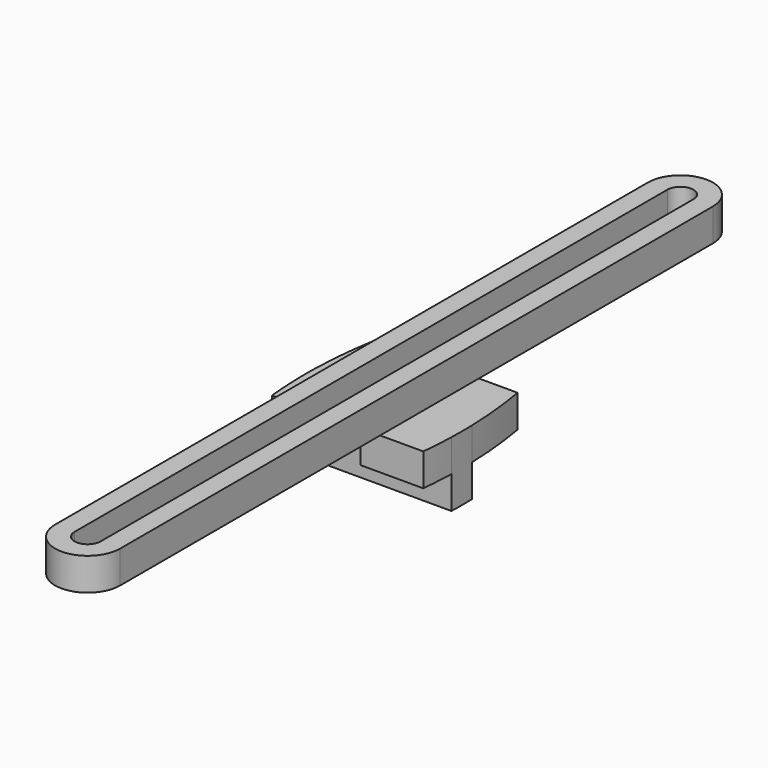
from build123d import *

# Parameters (mm, degrees)
F0_W     = 3
F0_H     = 10
F0_H_2   = 5
F1_DEPTH = 5
F2_START = -5
F2_DEPTH = 5
F3_DEPTH = 5


with BuildPart() as f1:
    # F0 (on Top) → F1 (new body)
    with BuildSketch(Plane.XY):
        with Locations((3.5, 7)):
            Rectangle(F0_W, F0_H)
        with BuildLine():
            Line((10.9485099174, 12), (5, 12))
            Line((5, 12), (5, 2))
            Line((5, 2), (11.9710084021, 2))
            ThreePointArc((11.9710084021, 2), (11.6421053306, 7.0186448683), (10.9485099174, 12))
        make_face()
        Polygon((5, 2), (2, 2), (2, -2), (5, -2), (5, 0), align=None)
        with BuildLine():
            Line((11.9710084021, 2), (5, 2))
            Line((5, 2), (5, 0))
            Line((5, 0), (5, -2))
            Line((5, -2), (11.9710084021, -2))
            ThreePointArc((11.9710084021, -2), (11.9927517198, -1.0001050586), (12, 0))
            ThreePointArc((12, 0), (11.9927517198, 1.0001050586), (11.9710084021, 2))
        make_face()
        with Locations((3.5, -4.5)):
            Rectangle(F0_W, F0_H_2)
        with BuildLine():
            Line((11.9710084021, -2), (5, -2))
            Line((5, -2), (5, -7))
            Line((5, -7), (11.6440092069, -7))
            ThreePointArc((11.6440092069, -7), (11.8529103806, -4.5029692558), (11.9710084021, -2))
        make_face()
    extrude(amount=-F1_DEPTH)



with BuildPart() as f1b:
    # F0 (on Top) → F1, piece 2 (new body)
    with BuildSketch(Plane.XY):
        with Locations((-3.5, 7)):
            Rectangle(F0_W, F0_H)
        with BuildLine():
            Line((-5, 2), (-5, 12))
            Line((-5, 12), (-10.9485099174, 12))
            ThreePointArc((-10.9485099174, 12), (-11.6421053306, 7.0186448683), (-11.9710084021, 2))
            Line((-11.9710084021, 2), (-5, 2))
        make_face()
        Polygon((-2, -2), (-2, 2), (-5, 2), (-5, 0), (-5, -2), align=None)
        with BuildLine():
            Line((-5, 0), (-5, 2))
            Line((-5, 2), (-11.9710084021, 2))
            ThreePointArc((-11.9710084021, 2), (-11.9927517198, 1.0001050586), (-12, 0))
            ThreePointArc((-12, 0), (-11.9927517198, -1.0001050586), (-11.9710084021, -2))
            Line((-11.9710084021, -2), (-5, -2))
            Line((-5, -2), (-5, 0))
        make_face()
        with Locations((-3.5, -4.5)):
            Rectangle(F0_W, F0_H_2)
        with BuildLine():
            Line((-5, -7), (-5, -2))
            Line((-5, -2), (-11.9710084021, -2))
            ThreePointArc((-11.9710084021, -2), (-11.8529103806, -4.5029692558), (-11.6440092069, -7))
            Line((-11.6440092069, -7), (-5, -7))
        make_face()
    extrude(amount=-F1_DEPTH)


with BuildPart() as f1_1:
    add(f1.part)

    add(f1b.part)  # F2 merges F1b
    # F0 (on Top) → F2 (join)
    with BuildSketch(Plane.XY.offset(F2_START)):
        Polygon((2, -2), (2, 2), (0, 2), (-2, 2), (-2, -2), (0, -2), align=None)
        Polygon((5, 2), (2, 2), (2, -2), (5, -2), (5, 0), align=None)
        Polygon((-2, -2), (-2, 2), (-5, 2), (-5, 0), (-5, -2), align=None)
        with BuildLine():
            Line((11.9710084021, 2), (5, 2))
            Line((5, 2), (5, 0))
            Line((5, 0), (5, -2))
            Line((5, -2), (11.9710084021, -2))
            ThreePointArc((11.9710084021, -2), (11.9927517198, -1.0001050586), (12, 0))
            ThreePointArc((12, 0), (11.9927517198, 1.0001050586), (11.9710084021, 2))
        make_face()
        with BuildLine():
            Line((-5, 0), (-5, 2))
            Line((-5, 2), (-11.9710084021, 2))
            ThreePointArc((-11.9710084021, 2), (-11.9927517198, 1.0001050586), (-12, 0))
            ThreePointArc((-12, 0), (-11.9927517198, -1.0001050586), (-11.9710084021, -2))
            Line((-11.9710084021, -2), (-5, -2))
            Line((-5, -2), (-5, 0))
        make_face()
    extrude(amount=-F2_DEPTH)

    # F0 (on Top) → F3 (join)
    with BuildSketch(Plane.XY):
        with BuildLine():
            ThreePointArc((-2, 57), (0, 59), (2, 57))
            Line((2, 57), (2, 12))
            Line((2, 12), (5, 12))
            Line((5, 12), (5, 57))
            ThreePointArc((5, 57), (0, 62), (-5, 57))
            Line((-5, 57), (-5, 12))
            Line((-5, 12), (-2, 12))
            Line((-2, 12), (-2, 57))
        make_face()
        with Locations((3.5, 7)):
            Rectangle(F0_W, F0_H)
        with Locations((-3.5, 7)):
            Rectangle(F0_W, F0_H)
        Polygon((5, 2), (2, 2), (2, -2), (5, -2), (5, 0), align=None)
        Polygon((-2, -2), (-2, 2), (-5, 2), (-5, 0), (-5, -2), align=None)
        with Locations((3.5, -4.5)):
            Rectangle(F0_W, F0_H_2)
        with Locations((-3.5, -4.5)):
            Rectangle(F0_W, F0_H_2)
        with BuildLine():
            Line((5, -7), (2, -7))
            Line((2, -7), (2, -57))
            ThreePointArc((2, -57), (0, -59), (-2, -57))
            Line((-2, -57), (-2, -7))
            Line((-2, -7), (-5, -7))
            Line((-5, -7), (-5, -57))
            ThreePointArc((-5, -57), (0, -62), (5, -57))
            Line((5, -57), (5, -7))
        make_face()
    extrude(amount=F3_DEPTH)


solid = f1_1.part
